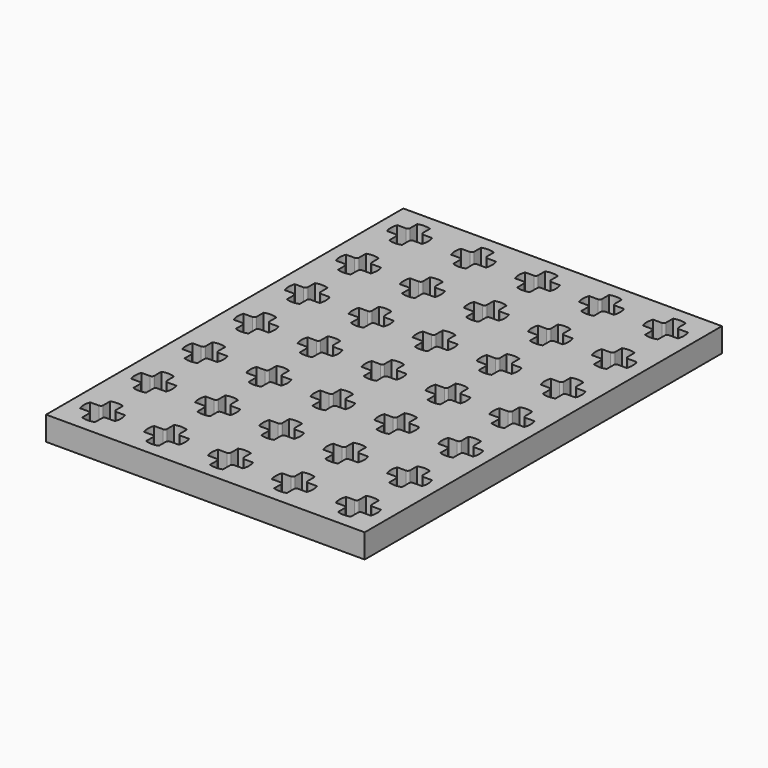
from build123d import *

# Parameters (mm, degrees)
F0_W     = 39.85
F0_H     = 55.85
F1_DEPTH = 3


# Not quite as in the source:
# - a feature names something its author has since deleted; it is built from what else it names


with BuildPart() as f1:
    # F0 (on Top) → F1 (new body)
    with BuildSketch(Plane.XY):
        Rectangle(F0_W, F0_H)
        with BuildLine():
            ThreePointArc((-15.2, -26.1830311496), (-16, -26.325), (-16.8, -26.1830311496))
            Line((-16.8, -26.1830311496), (-16.8, -25.1))
            ThreePointArc((-16.8, -25.1), (-16.8878679656, -24.8878679656), (-17.1, -24.8))
            Line((-17.1, -24.8), (-18.1830311496, -24.8))
            ThreePointArc((-18.1830311496, -24.8), (-18.325, -24), (-18.1830311496, -23.2))
            Line((-18.1830311496, -23.2), (-17.1, -23.2))
            ThreePointArc((-17.1, -23.2), (-16.8878679656, -23.1121320344), (-16.8, -22.9))
            Line((-16.8, -22.9), (-16.8, -21.8169688504))
            ThreePointArc((-16.8, -21.8169688504), (-16, -21.675), (-15.2, -21.8169688504))
            Line((-15.2, -21.8169688504), (-15.2, -22.9))
            ThreePointArc((-15.2, -22.9), (-15.1121320344, -23.1121320344), (-14.9, -23.2))
            Line((-14.9, -23.2), (-13.8169688504, -23.2))
            ThreePointArc((-13.8169688504, -23.2), (-13.675, -24), (-13.8169688504, -24.8))
            Line((-13.8169688504, -24.8), (-14.9, -24.8))
            ThreePointArc((-14.9, -24.8), (-15.1121320344, -24.8878679656), (-15.2, -25.1))
            Line((-15.2, -25.1), (-15.2, -26.1830311496))
        make_face(mode=Mode.SUBTRACT)
        with BuildLine():
            ThreePointArc((-7.2, -26.1830311496), (-8, -26.325), (-8.8, -26.1830311496))
            Line((-8.8, -26.1830311496), (-8.8, -25.1))
            ThreePointArc((-8.8, -25.1), (-8.8878679656, -24.8878679656), (-9.1, -24.8))
            Line((-9.1, -24.8), (-10.1830311496, -24.8))
            ThreePointArc((-10.1830311496, -24.8), (-10.325, -24), (-10.1830311496, -23.2))
            Line((-10.1830311496, -23.2), (-9.1, -23.2))
            ThreePointArc((-9.1, -23.2), (-8.8878679656, -23.1121320344), (-8.8, -22.9))
            Line((-8.8, -22.9), (-8.8, -21.8169688504))
            ThreePointArc((-8.8, -21.8169688504), (-8, -21.675), (-7.2, -21.8169688504))
            Line((-7.2, -21.8169688504), (-7.2, -22.9))
            ThreePointArc((-7.2, -22.9), (-7.1121320344, -23.1121320344), (-6.9, -23.2))
            Line((-6.9, -23.2), (-5.8169688504, -23.2))
            ThreePointArc((-5.8169688504, -23.2), (-5.675, -24), (-5.8169688504, -24.8))
            Line((-5.8169688504, -24.8), (-6.9, -24.8))
            ThreePointArc((-6.9, -24.8), (-7.1121320344, -24.8878679656), (-7.2, -25.1))
            Line((-7.2, -25.1), (-7.2, -26.1830311496))
        make_face(mode=Mode.SUBTRACT)
        with BuildLine():
            ThreePointArc((-15.2, -18.1830311496), (-16, -18.325), (-16.8, -18.1830311496))
            Line((-16.8, -18.1830311496), (-16.8, -17.1))
            ThreePointArc((-16.8, -17.1), (-16.8878679656, -16.8878679656), (-17.1, -16.8))
            Line((-17.1, -16.8), (-18.1830311496, -16.8))
            ThreePointArc((-18.1830311496, -16.8), (-18.325, -16), (-18.1830311496, -15.2))
            Line((-18.1830311496, -15.2), (-17.1, -15.2))
            ThreePointArc((-17.1, -15.2), (-16.8878679656, -15.1121320344), (-16.8, -14.9))
            Line((-16.8, -14.9), (-16.8, -13.8169688504))
            ThreePointArc((-16.8, -13.8169688504), (-16, -13.675), (-15.2, -13.8169688504))
            Line((-15.2, -13.8169688504), (-15.2, -14.9))
            ThreePointArc((-15.2, -14.9), (-15.1121320344, -15.1121320344), (-14.9, -15.2))
            Line((-14.9, -15.2), (-13.8169688504, -15.2))
            ThreePointArc((-13.8169688504, -15.2), (-13.675, -16), (-13.8169688504, -16.8))
            Line((-13.8169688504, -16.8), (-14.9, -16.8))
            ThreePointArc((-14.9, -16.8), (-15.1121320344, -16.8878679656), (-15.2, -17.1))
            Line((-15.2, -17.1), (-15.2, -18.1830311496))
        make_face(mode=Mode.SUBTRACT)
        with BuildLine():
            ThreePointArc((-15.2, -10.1830311496), (-16, -10.325), (-16.8, -10.1830311496))
            Line((-16.8, -10.1830311496), (-16.8, -9.1))
            ThreePointArc((-16.8, -9.1), (-16.8878679656, -8.8878679656), (-17.1, -8.8))
            Line((-17.1, -8.8), (-18.1830311496, -8.8))
            ThreePointArc((-18.1830311496, -8.8), (-18.325, -8), (-18.1830311496, -7.2))
            Line((-18.1830311496, -7.2), (-17.1, -7.2))
            ThreePointArc((-17.1, -7.2), (-16.8878679656, -7.1121320344), (-16.8, -6.9))
            Line((-16.8, -6.9), (-16.8, -5.8169688504))
            ThreePointArc((-16.8, -5.8169688504), (-16, -5.675), (-15.2, -5.8169688504))
            Line((-15.2, -5.8169688504), (-15.2, -6.9))
            ThreePointArc((-15.2, -6.9), (-15.1121320344, -7.1121320344), (-14.9, -7.2))
            Line((-14.9, -7.2), (-13.8169688504, -7.2))
            ThreePointArc((-13.8169688504, -7.2), (-13.675, -8), (-13.8169688504, -8.8))
            Line((-13.8169688504, -8.8), (-14.9, -8.8))
            ThreePointArc((-14.9, -8.8), (-15.1121320344, -8.8878679656), (-15.2, -9.1))
            Line((-15.2, -9.1), (-15.2, -10.1830311496))
        make_face(mode=Mode.SUBTRACT)
        with BuildLine():
            ThreePointArc((-7.2, -18.1830311496), (-8, -18.325), (-8.8, -18.1830311496))
            Line((-8.8, -18.1830311496), (-8.8, -17.1))
            ThreePointArc((-8.8, -17.1), (-8.8878679656, -16.8878679656), (-9.1, -16.8))
            Line((-9.1, -16.8), (-10.1830311496, -16.8))
            ThreePointArc((-10.1830311496, -16.8), (-10.325, -16), (-10.1830311496, -15.2))
            Line((-10.1830311496, -15.2), (-9.1, -15.2))
            ThreePointArc((-9.1, -15.2), (-8.8878679656, -15.1121320344), (-8.8, -14.9))
            Line((-8.8, -14.9), (-8.8, -13.8169688504))
            ThreePointArc((-8.8, -13.8169688504), (-8, -13.675), (-7.2, -13.8169688504))
            Line((-7.2, -13.8169688504), (-7.2, -14.9))
            ThreePointArc((-7.2, -14.9), (-7.1121320344, -15.1121320344), (-6.9, -15.2))
            Line((-6.9, -15.2), (-5.8169688504, -15.2))
            ThreePointArc((-5.8169688504, -15.2), (-5.675, -16), (-5.8169688504, -16.8))
            Line((-5.8169688504, -16.8), (-6.9, -16.8))
            ThreePointArc((-6.9, -16.8), (-7.1121320344, -16.8878679656), (-7.2, -17.1))
            Line((-7.2, -17.1), (-7.2, -18.1830311496))
        make_face(mode=Mode.SUBTRACT)
        with BuildLine():
            ThreePointArc((-7.2, -10.1830311496), (-8, -10.325), (-8.8, -10.1830311496))
            Line((-8.8, -10.1830311496), (-8.8, -9.1))
            ThreePointArc((-8.8, -9.1), (-8.8878679656, -8.8878679656), (-9.1, -8.8))
            Line((-9.1, -8.8), (-10.1830311496, -8.8))
            ThreePointArc((-10.1830311496, -8.8), (-10.325, -8), (-10.1830311496, -7.2))
            Line((-10.1830311496, -7.2), (-9.1, -7.2))
            ThreePointArc((-9.1, -7.2), (-8.8878679656, -7.1121320344), (-8.8, -6.9))
            Line((-8.8, -6.9), (-8.8, -5.8169688504))
            ThreePointArc((-8.8, -5.8169688504), (-8, -5.675), (-7.2, -5.8169688504))
            Line((-7.2, -5.8169688504), (-7.2, -6.9))
            ThreePointArc((-7.2, -6.9), (-7.1121320344, -7.1121320344), (-6.9, -7.2))
            Line((-6.9, -7.2), (-5.8169688504, -7.2))
            ThreePointArc((-5.8169688504, -7.2), (-5.675, -8), (-5.8169688504, -8.8))
            Line((-5.8169688504, -8.8), (-6.9, -8.8))
            ThreePointArc((-6.9, -8.8), (-7.1121320344, -8.8878679656), (-7.2, -9.1))
            Line((-7.2, -9.1), (-7.2, -10.1830311496))
        make_face(mode=Mode.SUBTRACT)
        with BuildLine():
            ThreePointArc((0.8, -26.1830311496), (0, -26.325), (-0.8, -26.1830311496))
            Line((-0.8, -26.1830311496), (-0.8, -25.1))
            ThreePointArc((-0.8, -25.1), (-0.8878679656, -24.8878679656), (-1.1, -24.8))
            Line((-1.1, -24.8), (-2.1830311496, -24.8))
            ThreePointArc((-2.1830311496, -24.8), (-2.325, -24), (-2.1830311496, -23.2))
            Line((-2.1830311496, -23.2), (-1.1, -23.2))
            ThreePointArc((-1.1, -23.2), (-0.8878679656, -23.1121320344), (-0.8, -22.9))
            Line((-0.8, -22.9), (-0.8, -21.8169688504))
            ThreePointArc((-0.8, -21.8169688504), (0, -21.675), (0.8, -21.8169688504))
            Line((0.8, -21.8169688504), (0.8, -22.9))
            ThreePointArc((0.8, -22.9), (0.8878679656, -23.1121320344), (1.1, -23.2))
            Line((1.1, -23.2), (2.1830311496, -23.2))
            ThreePointArc((2.1830311496, -23.2), (2.325, -24), (2.1830311496, -24.8))
            Line((2.1830311496, -24.8), (1.1, -24.8))
            ThreePointArc((1.1, -24.8), (0.8878679656, -24.8878679656), (0.8, -25.1))
            Line((0.8, -25.1), (0.8, -26.1830311496))
        make_face(mode=Mode.SUBTRACT)
        with BuildLine():
            ThreePointArc((8.8, -26.1830311496), (8, -26.325), (7.2, -26.1830311496))
            Line((7.2, -26.1830311496), (7.2, -25.1))
            ThreePointArc((7.2, -25.1), (7.1121320344, -24.8878679656), (6.9, -24.8))
            Line((6.9, -24.8), (5.8169688504, -24.8))
            ThreePointArc((5.8169688504, -24.8), (5.675, -24), (5.8169688504, -23.2))
            Line((5.8169688504, -23.2), (6.9, -23.2))
            ThreePointArc((6.9, -23.2), (7.1121320344, -23.1121320344), (7.2, -22.9))
            Line((7.2, -22.9), (7.2, -21.8169688504))
            ThreePointArc((7.2, -21.8169688504), (8, -21.675), (8.8, -21.8169688504))
            Line((8.8, -21.8169688504), (8.8, -22.9))
            ThreePointArc((8.8, -22.9), (8.8878679656, -23.1121320344), (9.1, -23.2))
            Line((9.1, -23.2), (10.1830311496, -23.2))
            ThreePointArc((10.1830311496, -23.2), (10.325, -24), (10.1830311496, -24.8))
            Line((10.1830311496, -24.8), (9.1, -24.8))
            ThreePointArc((9.1, -24.8), (8.8878679656, -24.8878679656), (8.8, -25.1))
            Line((8.8, -25.1), (8.8, -26.1830311496))
        make_face(mode=Mode.SUBTRACT)
        with BuildLine():
            ThreePointArc((16.8, -26.1830311496), (16, -26.325), (15.2, -26.1830311496))
            Line((15.2, -26.1830311496), (15.2, -25.1))
            ThreePointArc((15.2, -25.1), (15.1121320344, -24.8878679656), (14.9, -24.8))
            Line((14.9, -24.8), (13.8169688504, -24.8))
            ThreePointArc((13.8169688504, -24.8), (13.675, -24), (13.8169688504, -23.2))
            Line((13.8169688504, -23.2), (14.9, -23.2))
            ThreePointArc((14.9, -23.2), (15.1121320344, -23.1121320344), (15.2, -22.9))
            Line((15.2, -22.9), (15.2, -21.8169688504))
            ThreePointArc((15.2, -21.8169688504), (16, -21.675), (16.8, -21.8169688504))
            Line((16.8, -21.8169688504), (16.8, -22.9))
            ThreePointArc((16.8, -22.9), (16.8878679656, -23.1121320344), (17.1, -23.2))
            Line((17.1, -23.2), (18.1830311496, -23.2))
            ThreePointArc((18.1830311496, -23.2), (18.325, -24), (18.1830311496, -24.8))
            Line((18.1830311496, -24.8), (17.1, -24.8))
            ThreePointArc((17.1, -24.8), (16.8878679656, -24.8878679656), (16.8, -25.1))
            Line((16.8, -25.1), (16.8, -26.1830311496))
        make_face(mode=Mode.SUBTRACT)
        with BuildLine():
            ThreePointArc((0.8, -18.1830311496), (0, -18.325), (-0.8, -18.1830311496))
            Line((-0.8, -18.1830311496), (-0.8, -17.1))
            ThreePointArc((-0.8, -17.1), (-0.8878679656, -16.8878679656), (-1.1, -16.8))
            Line((-1.1, -16.8), (-2.1830311496, -16.8))
            ThreePointArc((-2.1830311496, -16.8), (-2.325, -16), (-2.1830311496, -15.2))
            Line((-2.1830311496, -15.2), (-1.1, -15.2))
            ThreePointArc((-1.1, -15.2), (-0.8878679656, -15.1121320344), (-0.8, -14.9))
            Line((-0.8, -14.9), (-0.8, -13.8169688504))
            ThreePointArc((-0.8, -13.8169688504), (0, -13.675), (0.8, -13.8169688504))
            Line((0.8, -13.8169688504), (0.8, -14.9))
            ThreePointArc((0.8, -14.9), (0.8878679656, -15.1121320344), (1.1, -15.2))
            Line((1.1, -15.2), (2.1830311496, -15.2))
            ThreePointArc((2.1830311496, -15.2), (2.325, -16), (2.1830311496, -16.8))
            Line((2.1830311496, -16.8), (1.1, -16.8))
            ThreePointArc((1.1, -16.8), (0.8878679656, -16.8878679656), (0.8, -17.1))
            Line((0.8, -17.1), (0.8, -18.1830311496))
        make_face(mode=Mode.SUBTRACT)
        with BuildLine():
            ThreePointArc((8.8, -18.1830311496), (8, -18.325), (7.2, -18.1830311496))
            Line((7.2, -18.1830311496), (7.2, -17.1))
            ThreePointArc((7.2, -17.1), (7.1121320344, -16.8878679656), (6.9, -16.8))
            Line((6.9, -16.8), (5.8169688504, -16.8))
            ThreePointArc((5.8169688504, -16.8), (5.675, -16), (5.8169688504, -15.2))
            Line((5.8169688504, -15.2), (6.9, -15.2))
            ThreePointArc((6.9, -15.2), (7.1121320344, -15.1121320344), (7.2, -14.9))
            Line((7.2, -14.9), (7.2, -13.8169688504))
            ThreePointArc((7.2, -13.8169688504), (8, -13.675), (8.8, -13.8169688504))
            Line((8.8, -13.8169688504), (8.8, -14.9))
            ThreePointArc((8.8, -14.9), (8.8878679656, -15.1121320344), (9.1, -15.2))
            Line((9.1, -15.2), (10.1830311496, -15.2))
            ThreePointArc((10.1830311496, -15.2), (10.325, -16), (10.1830311496, -16.8))
            Line((10.1830311496, -16.8), (9.1, -16.8))
            ThreePointArc((9.1, -16.8), (8.8878679656, -16.8878679656), (8.8, -17.1))
            Line((8.8, -17.1), (8.8, -18.1830311496))
        make_face(mode=Mode.SUBTRACT)
        with BuildLine():
            ThreePointArc((0.8, -10.1830311496), (0, -10.325), (-0.8, -10.1830311496))
            Line((-0.8, -10.1830311496), (-0.8, -9.1))
            ThreePointArc((-0.8, -9.1), (-0.8878679656, -8.8878679656), (-1.1, -8.8))
            Line((-1.1, -8.8), (-2.1830311496, -8.8))
            ThreePointArc((-2.1830311496, -8.8), (-2.325, -8), (-2.1830311496, -7.2))
            Line((-2.1830311496, -7.2), (-1.1, -7.2))
            ThreePointArc((-1.1, -7.2), (-0.8878679656, -7.1121320344), (-0.8, -6.9))
            Line((-0.8, -6.9), (-0.8, -5.8169688504))
            ThreePointArc((-0.8, -5.8169688504), (0, -5.675), (0.8, -5.8169688504))
            Line((0.8, -5.8169688504), (0.8, -6.9))
            ThreePointArc((0.8, -6.9), (0.8878679656, -7.1121320344), (1.1, -7.2))
            Line((1.1, -7.2), (2.1830311496, -7.2))
            ThreePointArc((2.1830311496, -7.2), (2.325, -8), (2.1830311496, -8.8))
            Line((2.1830311496, -8.8), (1.1, -8.8))
            ThreePointArc((1.1, -8.8), (0.8878679656, -8.8878679656), (0.8, -9.1))
            Line((0.8, -9.1), (0.8, -10.1830311496))
        make_face(mode=Mode.SUBTRACT)
        with BuildLine():
            ThreePointArc((8.8, -10.1830311496), (8, -10.325), (7.2, -10.1830311496))
            Line((7.2, -10.1830311496), (7.2, -9.1))
            ThreePointArc((7.2, -9.1), (7.1121320344, -8.8878679656), (6.9, -8.8))
            Line((6.9, -8.8), (5.8169688504, -8.8))
            ThreePointArc((5.8169688504, -8.8), (5.675, -8), (5.8169688504, -7.2))
            Line((5.8169688504, -7.2), (6.9, -7.2))
            ThreePointArc((6.9, -7.2), (7.1121320344, -7.1121320344), (7.2, -6.9))
            Line((7.2, -6.9), (7.2, -5.8169688504))
            ThreePointArc((7.2, -5.8169688504), (8, -5.675), (8.8, -5.8169688504))
            Line((8.8, -5.8169688504), (8.8, -6.9))
            ThreePointArc((8.8, -6.9), (8.8878679656, -7.1121320344), (9.1, -7.2))
            Line((9.1, -7.2), (10.1830311496, -7.2))
            ThreePointArc((10.1830311496, -7.2), (10.325, -8), (10.1830311496, -8.8))
            Line((10.1830311496, -8.8), (9.1, -8.8))
            ThreePointArc((9.1, -8.8), (8.8878679656, -8.8878679656), (8.8, -9.1))
            Line((8.8, -9.1), (8.8, -10.1830311496))
        make_face(mode=Mode.SUBTRACT)
        with BuildLine():
            ThreePointArc((16.8, -18.1830311496), (16, -18.325), (15.2, -18.1830311496))
            Line((15.2, -18.1830311496), (15.2, -17.1))
            ThreePointArc((15.2, -17.1), (15.1121320344, -16.8878679656), (14.9, -16.8))
            Line((14.9, -16.8), (13.8169688504, -16.8))
            ThreePointArc((13.8169688504, -16.8), (13.675, -16), (13.8169688504, -15.2))
            Line((13.8169688504, -15.2), (14.9, -15.2))
            ThreePointArc((14.9, -15.2), (15.1121320344, -15.1121320344), (15.2, -14.9))
            Line((15.2, -14.9), (15.2, -13.8169688504))
            ThreePointArc((15.2, -13.8169688504), (16, -13.675), (16.8, -13.8169688504))
            Line((16.8, -13.8169688504), (16.8, -14.9))
            ThreePointArc((16.8, -14.9), (16.8878679656, -15.1121320344), (17.1, -15.2))
            Line((17.1, -15.2), (18.1830311496, -15.2))
            ThreePointArc((18.1830311496, -15.2), (18.325, -16), (18.1830311496, -16.8))
            Line((18.1830311496, -16.8), (17.1, -16.8))
            ThreePointArc((17.1, -16.8), (16.8878679656, -16.8878679656), (16.8, -17.1))
            Line((16.8, -17.1), (16.8, -18.1830311496))
        make_face(mode=Mode.SUBTRACT)
        with BuildLine():
            ThreePointArc((16.8, -10.1830311496), (16, -10.325), (15.2, -10.1830311496))
            Line((15.2, -10.1830311496), (15.2, -9.1))
            ThreePointArc((15.2, -9.1), (15.1121320344, -8.8878679656), (14.9, -8.8))
            Line((14.9, -8.8), (13.8169688504, -8.8))
            ThreePointArc((13.8169688504, -8.8), (13.675, -8), (13.8169688504, -7.2))
            Line((13.8169688504, -7.2), (14.9, -7.2))
            ThreePointArc((14.9, -7.2), (15.1121320344, -7.1121320344), (15.2, -6.9))
            Line((15.2, -6.9), (15.2, -5.8169688504))
            ThreePointArc((15.2, -5.8169688504), (16, -5.675), (16.8, -5.8169688504))
            Line((16.8, -5.8169688504), (16.8, -6.9))
            ThreePointArc((16.8, -6.9), (16.8878679656, -7.1121320344), (17.1, -7.2))
            Line((17.1, -7.2), (18.1830311496, -7.2))
            ThreePointArc((18.1830311496, -7.2), (18.325, -8), (18.1830311496, -8.8))
            Line((18.1830311496, -8.8), (17.1, -8.8))
            ThreePointArc((17.1, -8.8), (16.8878679656, -8.8878679656), (16.8, -9.1))
            Line((16.8, -9.1), (16.8, -10.1830311496))
        make_face(mode=Mode.SUBTRACT)
        with BuildLine():
            ThreePointArc((-15.2, -2.1830311496), (-16, -2.325), (-16.8, -2.1830311496))
            Line((-16.8, -2.1830311496), (-16.8, -1.1))
            ThreePointArc((-16.8, -1.1), (-16.8878679656, -0.8878679656), (-17.1, -0.8))
            Line((-17.1, -0.8), (-18.1830311496, -0.8))
            ThreePointArc((-18.1830311496, -0.8), (-18.325, 0), (-18.1830311496, 0.8))
            Line((-18.1830311496, 0.8), (-17.1, 0.8))
            ThreePointArc((-17.1, 0.8), (-16.8878679656, 0.8878679656), (-16.8, 1.1))
            Line((-16.8, 1.1), (-16.8, 2.1830311496))
            ThreePointArc((-16.8, 2.1830311496), (-16, 2.325), (-15.2, 2.1830311496))
            Line((-15.2, 2.1830311496), (-15.2, 1.1))
            ThreePointArc((-15.2, 1.1), (-15.1121320344, 0.8878679656), (-14.9, 0.8))
            Line((-14.9, 0.8), (-13.8169688504, 0.8))
            ThreePointArc((-13.8169688504, 0.8), (-13.675, 0), (-13.8169688504, -0.8))
            Line((-13.8169688504, -0.8), (-14.9, -0.8))
            ThreePointArc((-14.9, -0.8), (-15.1121320344, -0.8878679656), (-15.2, -1.1))
            Line((-15.2, -1.1), (-15.2, -2.1830311496))
        make_face(mode=Mode.SUBTRACT)
        with BuildLine():
            ThreePointArc((-15.2, 5.8169688504), (-16, 5.675), (-16.8, 5.8169688504))
            Line((-16.8, 5.8169688504), (-16.8, 6.9))
            ThreePointArc((-16.8, 6.9), (-16.8878679656, 7.1121320344), (-17.1, 7.2))
            Line((-17.1, 7.2), (-18.1830311496, 7.2))
            ThreePointArc((-18.1830311496, 7.2), (-18.325, 8), (-18.1830311496, 8.8))
            Line((-18.1830311496, 8.8), (-17.1, 8.8))
            ThreePointArc((-17.1, 8.8), (-16.8878679656, 8.8878679656), (-16.8, 9.1))
            Line((-16.8, 9.1), (-16.8, 10.1830311496))
            ThreePointArc((-16.8, 10.1830311496), (-16, 10.325), (-15.2, 10.1830311496))
            Line((-15.2, 10.1830311496), (-15.2, 9.1))
            ThreePointArc((-15.2, 9.1), (-15.1121320344, 8.8878679656), (-14.9, 8.8))
            Line((-14.9, 8.8), (-13.8169688504, 8.8))
            ThreePointArc((-13.8169688504, 8.8), (-13.675, 8), (-13.8169688504, 7.2))
            Line((-13.8169688504, 7.2), (-14.9, 7.2))
            ThreePointArc((-14.9, 7.2), (-15.1121320344, 7.1121320344), (-15.2, 6.9))
            Line((-15.2, 6.9), (-15.2, 5.8169688504))
        make_face(mode=Mode.SUBTRACT)
        with BuildLine():
            ThreePointArc((-7.2, -2.1830311496), (-8, -2.325), (-8.8, -2.1830311496))
            Line((-8.8, -2.1830311496), (-8.8, -1.1))
            ThreePointArc((-8.8, -1.1), (-8.8878679656, -0.8878679656), (-9.1, -0.8))
            Line((-9.1, -0.8), (-10.1830311496, -0.8))
            ThreePointArc((-10.1830311496, -0.8), (-10.325, 0), (-10.1830311496, 0.8))
            Line((-10.1830311496, 0.8), (-9.1, 0.8))
            ThreePointArc((-9.1, 0.8), (-8.8878679656, 0.8878679656), (-8.8, 1.1))
            Line((-8.8, 1.1), (-8.8, 2.1830311496))
            ThreePointArc((-8.8, 2.1830311496), (-8, 2.325), (-7.2, 2.1830311496))
            Line((-7.2, 2.1830311496), (-7.2, 1.1))
            ThreePointArc((-7.2, 1.1), (-7.1121320344, 0.8878679656), (-6.9, 0.8))
            Line((-6.9, 0.8), (-5.8169688504, 0.8))
            ThreePointArc((-5.8169688504, 0.8), (-5.675, 0), (-5.8169688504, -0.8))
            Line((-5.8169688504, -0.8), (-6.9, -0.8))
            ThreePointArc((-6.9, -0.8), (-7.1121320344, -0.8878679656), (-7.2, -1.1))
            Line((-7.2, -1.1), (-7.2, -2.1830311496))
        make_face(mode=Mode.SUBTRACT)
        with BuildLine():
            ThreePointArc((-7.2, 5.8169688504), (-8, 5.675), (-8.8, 5.8169688504))
            Line((-8.8, 5.8169688504), (-8.8, 6.9))
            ThreePointArc((-8.8, 6.9), (-8.8878679656, 7.1121320344), (-9.1, 7.2))
            Line((-9.1, 7.2), (-10.1830311496, 7.2))
            ThreePointArc((-10.1830311496, 7.2), (-10.325, 8), (-10.1830311496, 8.8))
            Line((-10.1830311496, 8.8), (-9.1, 8.8))
            ThreePointArc((-9.1, 8.8), (-8.8878679656, 8.8878679656), (-8.8, 9.1))
            Line((-8.8, 9.1), (-8.8, 10.1830311496))
            ThreePointArc((-8.8, 10.1830311496), (-8, 10.325), (-7.2, 10.1830311496))
            Line((-7.2, 10.1830311496), (-7.2, 9.1))
            ThreePointArc((-7.2, 9.1), (-7.1121320344, 8.8878679656), (-6.9, 8.8))
            Line((-6.9, 8.8), (-5.8169688504, 8.8))
            ThreePointArc((-5.8169688504, 8.8), (-5.675, 8), (-5.8169688504, 7.2))
            Line((-5.8169688504, 7.2), (-6.9, 7.2))
            ThreePointArc((-6.9, 7.2), (-7.1121320344, 7.1121320344), (-7.2, 6.9))
            Line((-7.2, 6.9), (-7.2, 5.8169688504))
        make_face(mode=Mode.SUBTRACT)
        with BuildLine():
            ThreePointArc((-15.2, 13.8169688504), (-16, 13.675), (-16.8, 13.8169688504))
            Line((-16.8, 13.8169688504), (-16.8, 14.9))
            ThreePointArc((-16.8, 14.9), (-16.8878679656, 15.1121320344), (-17.1, 15.2))
            Line((-17.1, 15.2), (-18.1830311496, 15.2))
            ThreePointArc((-18.1830311496, 15.2), (-18.325, 16), (-18.1830311496, 16.8))
            Line((-18.1830311496, 16.8), (-17.1, 16.8))
            ThreePointArc((-17.1, 16.8), (-16.8878679656, 16.8878679656), (-16.8, 17.1))
            Line((-16.8, 17.1), (-16.8, 18.1830311496))
            ThreePointArc((-16.8, 18.1830311496), (-16, 18.325), (-15.2, 18.1830311496))
            Line((-15.2, 18.1830311496), (-15.2, 17.1))
            ThreePointArc((-15.2, 17.1), (-15.1121320344, 16.8878679656), (-14.9, 16.8))
            Line((-14.9, 16.8), (-13.8169688504, 16.8))
            ThreePointArc((-13.8169688504, 16.8), (-13.675, 16), (-13.8169688504, 15.2))
            Line((-13.8169688504, 15.2), (-14.9, 15.2))
            ThreePointArc((-14.9, 15.2), (-15.1121320344, 15.1121320344), (-15.2, 14.9))
            Line((-15.2, 14.9), (-15.2, 13.8169688504))
        make_face(mode=Mode.SUBTRACT)
        with BuildLine():
            ThreePointArc((-16.8, 26.1830311496), (-16, 26.325), (-15.2, 26.1830311496))
            Line((-15.2, 26.1830311496), (-15.2, 25.1))
            ThreePointArc((-15.2, 25.1), (-15.1121320344, 24.8878679656), (-14.9, 24.8))
            Line((-14.9, 24.8), (-13.8169688504, 24.8))
            ThreePointArc((-13.8169688504, 24.8), (-13.675, 24), (-13.8169688504, 23.2))
            Line((-13.8169688504, 23.2), (-14.9, 23.2))
            ThreePointArc((-14.9, 23.2), (-15.1121320344, 23.1121320344), (-15.2, 22.9))
            Line((-15.2, 22.9), (-15.2, 21.8169688504))
            ThreePointArc((-15.2, 21.8169688504), (-16, 21.675), (-16.8, 21.8169688504))
            Line((-16.8, 21.8169688504), (-16.8, 22.9))
            ThreePointArc((-16.8, 22.9), (-16.8878679656, 23.1121320344), (-17.1, 23.2))
            Line((-17.1, 23.2), (-18.1830311496, 23.2))
            ThreePointArc((-18.1830311496, 23.2), (-18.325, 24), (-18.1830311496, 24.8))
            Line((-18.1830311496, 24.8), (-17.1, 24.8))
            ThreePointArc((-17.1, 24.8), (-16.8878679656, 24.8878679656), (-16.8, 25.1))
            Line((-16.8, 25.1), (-16.8, 26.1830311496))
        make_face(mode=Mode.SUBTRACT)
        with BuildLine():
            ThreePointArc((-7.2, 13.8169688504), (-8, 13.675), (-8.8, 13.8169688504))
            Line((-8.8, 13.8169688504), (-8.8, 14.9))
            ThreePointArc((-8.8, 14.9), (-8.8878679656, 15.1121320344), (-9.1, 15.2))
            Line((-9.1, 15.2), (-10.1830311496, 15.2))
            ThreePointArc((-10.1830311496, 15.2), (-10.325, 16), (-10.1830311496, 16.8))
            Line((-10.1830311496, 16.8), (-9.1, 16.8))
            ThreePointArc((-9.1, 16.8), (-8.8878679656, 16.8878679656), (-8.8, 17.1))
            Line((-8.8, 17.1), (-8.8, 18.1830311496))
            ThreePointArc((-8.8, 18.1830311496), (-8, 18.325), (-7.2, 18.1830311496))
            Line((-7.2, 18.1830311496), (-7.2, 17.1))
            ThreePointArc((-7.2, 17.1), (-7.1121320344, 16.8878679656), (-6.9, 16.8))
            Line((-6.9, 16.8), (-5.8169688504, 16.8))
            ThreePointArc((-5.8169688504, 16.8), (-5.675, 16), (-5.8169688504, 15.2))
            Line((-5.8169688504, 15.2), (-6.9, 15.2))
            ThreePointArc((-6.9, 15.2), (-7.1121320344, 15.1121320344), (-7.2, 14.9))
            Line((-7.2, 14.9), (-7.2, 13.8169688504))
        make_face(mode=Mode.SUBTRACT)
        with BuildLine():
            ThreePointArc((-7.2, 21.8169688504), (-8, 21.675), (-8.8, 21.8169688504))
            Line((-8.8, 21.8169688504), (-8.8, 22.9))
            ThreePointArc((-8.8, 22.9), (-8.8878679656, 23.1121320344), (-9.1, 23.2))
            Line((-9.1, 23.2), (-10.1830311496, 23.2))
            ThreePointArc((-10.1830311496, 23.2), (-10.325, 24), (-10.1830311496, 24.8))
            Line((-10.1830311496, 24.8), (-9.1, 24.8))
            ThreePointArc((-9.1, 24.8), (-8.8878679656, 24.8878679656), (-8.8, 25.1))
            Line((-8.8, 25.1), (-8.8, 26.1830311496))
            ThreePointArc((-8.8, 26.1830311496), (-8, 26.325), (-7.2, 26.1830311496))
            Line((-7.2, 26.1830311496), (-7.2, 25.1))
            ThreePointArc((-7.2, 25.1), (-7.1121320344, 24.8878679656), (-6.9, 24.8))
            Line((-6.9, 24.8), (-5.8169688504, 24.8))
            ThreePointArc((-5.8169688504, 24.8), (-5.675, 24), (-5.8169688504, 23.2))
            Line((-5.8169688504, 23.2), (-6.9, 23.2))
            ThreePointArc((-6.9, 23.2), (-7.1121320344, 23.1121320344), (-7.2, 22.9))
            Line((-7.2, 22.9), (-7.2, 21.8169688504))
        make_face(mode=Mode.SUBTRACT)
        with BuildLine():
            ThreePointArc((0.8, -2.1830311496), (0, -2.325), (-0.8, -2.1830311496))
            Line((-0.8, -2.1830311496), (-0.8, -1.1))
            ThreePointArc((-0.8, -1.1), (-0.8878679656, -0.8878679656), (-1.1, -0.8))
            Line((-1.1, -0.8), (-2.1830311496, -0.8))
            ThreePointArc((-2.1830311496, -0.8), (-2.325, 0), (-2.1830311496, 0.8))
            Line((-2.1830311496, 0.8), (-1.1, 0.8))
            ThreePointArc((-1.1, 0.8), (-0.8878679656, 0.8878679656), (-0.8, 1.1))
            Line((-0.8, 1.1), (-0.8, 2.1830311496))
            ThreePointArc((-0.8, 2.1830311496), (0, 2.325), (0.8, 2.1830311496))
            Line((0.8, 2.1830311496), (0.8, 1.1))
            ThreePointArc((0.8, 1.1), (0.8878679656, 0.8878679656), (1.1, 0.8))
            Line((1.1, 0.8), (2.1830311496, 0.8))
            ThreePointArc((2.1830311496, 0.8), (2.325, 0), (2.1830311496, -0.8))
            Line((2.1830311496, -0.8), (1.1, -0.8))
            ThreePointArc((1.1, -0.8), (0.8878679656, -0.8878679656), (0.8, -1.1))
            Line((0.8, -1.1), (0.8, -2.1830311496))
        make_face(mode=Mode.SUBTRACT)
        with BuildLine():
            ThreePointArc((8.8, -2.1830311496), (8, -2.325), (7.2, -2.1830311496))
            Line((7.2, -2.1830311496), (7.2, -1.1))
            ThreePointArc((7.2, -1.1), (7.1121320344, -0.8878679656), (6.9, -0.8))
            Line((6.9, -0.8), (5.8169688504, -0.8))
            ThreePointArc((5.8169688504, -0.8), (5.675, 0), (5.8169688504, 0.8))
            Line((5.8169688504, 0.8), (6.9, 0.8))
            ThreePointArc((6.9, 0.8), (7.1121320344, 0.8878679656), (7.2, 1.1))
            Line((7.2, 1.1), (7.2, 2.1830311496))
            ThreePointArc((7.2, 2.1830311496), (8, 2.325), (8.8, 2.1830311496))
            Line((8.8, 2.1830311496), (8.8, 1.1))
            ThreePointArc((8.8, 1.1), (8.8878679656, 0.8878679656), (9.1, 0.8))
            Line((9.1, 0.8), (10.1830311496, 0.8))
            ThreePointArc((10.1830311496, 0.8), (10.325, 0), (10.1830311496, -0.8))
            Line((10.1830311496, -0.8), (9.1, -0.8))
            ThreePointArc((9.1, -0.8), (8.8878679656, -0.8878679656), (8.8, -1.1))
            Line((8.8, -1.1), (8.8, -2.1830311496))
        make_face(mode=Mode.SUBTRACT)
        with BuildLine():
            ThreePointArc((0.8, 5.8169688504), (0, 5.675), (-0.8, 5.8169688504))
            Line((-0.8, 5.8169688504), (-0.8, 6.9))
            ThreePointArc((-0.8, 6.9), (-0.8878679656, 7.1121320344), (-1.1, 7.2))
            Line((-1.1, 7.2), (-2.1830311496, 7.2))
            ThreePointArc((-2.1830311496, 7.2), (-2.325, 8), (-2.1830311496, 8.8))
            Line((-2.1830311496, 8.8), (-1.1, 8.8))
            ThreePointArc((-1.1, 8.8), (-0.8878679656, 8.8878679656), (-0.8, 9.1))
            Line((-0.8, 9.1), (-0.8, 10.1830311496))
            ThreePointArc((-0.8, 10.1830311496), (0, 10.325), (0.8, 10.1830311496))
            Line((0.8, 10.1830311496), (0.8, 9.1))
            ThreePointArc((0.8, 9.1), (0.8878679656, 8.8878679656), (1.1, 8.8))
            Line((1.1, 8.8), (2.1830311496, 8.8))
            ThreePointArc((2.1830311496, 8.8), (2.325, 8), (2.1830311496, 7.2))
            Line((2.1830311496, 7.2), (1.1, 7.2))
            ThreePointArc((1.1, 7.2), (0.8878679656, 7.1121320344), (0.8, 6.9))
            Line((0.8, 6.9), (0.8, 5.8169688504))
        make_face(mode=Mode.SUBTRACT)
        with BuildLine():
            ThreePointArc((8.8, 5.8169688504), (8, 5.675), (7.2, 5.8169688504))
            Line((7.2, 5.8169688504), (7.2, 6.9))
            ThreePointArc((7.2, 6.9), (7.1121320344, 7.1121320344), (6.9, 7.2))
            Line((6.9, 7.2), (5.8169688504, 7.2))
            ThreePointArc((5.8169688504, 7.2), (5.675, 8), (5.8169688504, 8.8))
            Line((5.8169688504, 8.8), (6.9, 8.8))
            ThreePointArc((6.9, 8.8), (7.1121320344, 8.8878679656), (7.2, 9.1))
            Line((7.2, 9.1), (7.2, 10.1830311496))
            ThreePointArc((7.2, 10.1830311496), (8, 10.325), (8.8, 10.1830311496))
            Line((8.8, 10.1830311496), (8.8, 9.1))
            ThreePointArc((8.8, 9.1), (8.8878679656, 8.8878679656), (9.1, 8.8))
            Line((9.1, 8.8), (10.1830311496, 8.8))
            ThreePointArc((10.1830311496, 8.8), (10.325, 8), (10.1830311496, 7.2))
            Line((10.1830311496, 7.2), (9.1, 7.2))
            ThreePointArc((9.1, 7.2), (8.8878679656, 7.1121320344), (8.8, 6.9))
            Line((8.8, 6.9), (8.8, 5.8169688504))
        make_face(mode=Mode.SUBTRACT)
        with BuildLine():
            ThreePointArc((16.8, -2.1830311496), (16, -2.325), (15.2, -2.1830311496))
            Line((15.2, -2.1830311496), (15.2, -1.1))
            ThreePointArc((15.2, -1.1), (15.1121320344, -0.8878679656), (14.9, -0.8))
            Line((14.9, -0.8), (13.8169688504, -0.8))
            ThreePointArc((13.8169688504, -0.8), (13.675, 0), (13.8169688504, 0.8))
            Line((13.8169688504, 0.8), (14.9, 0.8))
            ThreePointArc((14.9, 0.8), (15.1121320344, 0.8878679656), (15.2, 1.1))
            Line((15.2, 1.1), (15.2, 2.1830311496))
            ThreePointArc((15.2, 2.1830311496), (16, 2.325), (16.8, 2.1830311496))
            Line((16.8, 2.1830311496), (16.8, 1.1))
            ThreePointArc((16.8, 1.1), (16.8878679656, 0.8878679656), (17.1, 0.8))
            Line((17.1, 0.8), (18.1830311496, 0.8))
            ThreePointArc((18.1830311496, 0.8), (18.325, 0), (18.1830311496, -0.8))
            Line((18.1830311496, -0.8), (17.1, -0.8))
            ThreePointArc((17.1, -0.8), (16.8878679656, -0.8878679656), (16.8, -1.1))
            Line((16.8, -1.1), (16.8, -2.1830311496))
        make_face(mode=Mode.SUBTRACT)
        with BuildLine():
            ThreePointArc((16.8, 5.8169688504), (16, 5.675), (15.2, 5.8169688504))
            Line((15.2, 5.8169688504), (15.2, 6.9))
            ThreePointArc((15.2, 6.9), (15.1121320344, 7.1121320344), (14.9, 7.2))
            Line((14.9, 7.2), (13.8169688504, 7.2))
            ThreePointArc((13.8169688504, 7.2), (13.675, 8), (13.8169688504, 8.8))
            Line((13.8169688504, 8.8), (14.9, 8.8))
            ThreePointArc((14.9, 8.8), (15.1121320344, 8.8878679656), (15.2, 9.1))
            Line((15.2, 9.1), (15.2, 10.1830311496))
            ThreePointArc((15.2, 10.1830311496), (16, 10.325), (16.8, 10.1830311496))
            Line((16.8, 10.1830311496), (16.8, 9.1))
            ThreePointArc((16.8, 9.1), (16.8878679656, 8.8878679656), (17.1, 8.8))
            Line((17.1, 8.8), (18.1830311496, 8.8))
            ThreePointArc((18.1830311496, 8.8), (18.325, 8), (18.1830311496, 7.2))
            Line((18.1830311496, 7.2), (17.1, 7.2))
            ThreePointArc((17.1, 7.2), (16.8878679656, 7.1121320344), (16.8, 6.9))
            Line((16.8, 6.9), (16.8, 5.8169688504))
        make_face(mode=Mode.SUBTRACT)
        with BuildLine():
            ThreePointArc((0.8, 13.8169688504), (0, 13.675), (-0.8, 13.8169688504))
            Line((-0.8, 13.8169688504), (-0.8, 14.9))
            ThreePointArc((-0.8, 14.9), (-0.8878679656, 15.1121320344), (-1.1, 15.2))
            Line((-1.1, 15.2), (-2.1830311496, 15.2))
            ThreePointArc((-2.1830311496, 15.2), (-2.325, 16), (-2.1830311496, 16.8))
            Line((-2.1830311496, 16.8), (-1.1, 16.8))
            ThreePointArc((-1.1, 16.8), (-0.8878679656, 16.8878679656), (-0.8, 17.1))
            Line((-0.8, 17.1), (-0.8, 18.1830311496))
            ThreePointArc((-0.8, 18.1830311496), (0, 18.325), (0.8, 18.1830311496))
            Line((0.8, 18.1830311496), (0.8, 17.1))
            ThreePointArc((0.8, 17.1), (0.8878679656, 16.8878679656), (1.1, 16.8))
            Line((1.1, 16.8), (2.1830311496, 16.8))
            ThreePointArc((2.1830311496, 16.8), (2.325, 16), (2.1830311496, 15.2))
            Line((2.1830311496, 15.2), (1.1, 15.2))
            ThreePointArc((1.1, 15.2), (0.8878679656, 15.1121320344), (0.8, 14.9))
            Line((0.8, 14.9), (0.8, 13.8169688504))
        make_face(mode=Mode.SUBTRACT)
        with BuildLine():
            ThreePointArc((8.8, 13.8169688504), (8, 13.675), (7.2, 13.8169688504))
            Line((7.2, 13.8169688504), (7.2, 14.9))
            ThreePointArc((7.2, 14.9), (7.1121320344, 15.1121320344), (6.9, 15.2))
            Line((6.9, 15.2), (5.8169688504, 15.2))
            ThreePointArc((5.8169688504, 15.2), (5.675, 16), (5.8169688504, 16.8))
            Line((5.8169688504, 16.8), (6.9, 16.8))
            ThreePointArc((6.9, 16.8), (7.1121320344, 16.8878679656), (7.2, 17.1))
            Line((7.2, 17.1), (7.2, 18.1830311496))
            ThreePointArc((7.2, 18.1830311496), (8, 18.325), (8.8, 18.1830311496))
            Line((8.8, 18.1830311496), (8.8, 17.1))
            ThreePointArc((8.8, 17.1), (8.8878679656, 16.8878679656), (9.1, 16.8))
            Line((9.1, 16.8), (10.1830311496, 16.8))
            ThreePointArc((10.1830311496, 16.8), (10.325, 16), (10.1830311496, 15.2))
            Line((10.1830311496, 15.2), (9.1, 15.2))
            ThreePointArc((9.1, 15.2), (8.8878679656, 15.1121320344), (8.8, 14.9))
            Line((8.8, 14.9), (8.8, 13.8169688504))
        make_face(mode=Mode.SUBTRACT)
        with BuildLine():
            ThreePointArc((0.8, 21.8169688504), (0, 21.675), (-0.8, 21.8169688504))
            Line((-0.8, 21.8169688504), (-0.8, 22.9))
            ThreePointArc((-0.8, 22.9), (-0.8878679656, 23.1121320344), (-1.1, 23.2))
            Line((-1.1, 23.2), (-2.1830311496, 23.2))
            ThreePointArc((-2.1830311496, 23.2), (-2.325, 24), (-2.1830311496, 24.8))
            Line((-2.1830311496, 24.8), (-1.1, 24.8))
            ThreePointArc((-1.1, 24.8), (-0.8878679656, 24.8878679656), (-0.8, 25.1))
            Line((-0.8, 25.1), (-0.8, 26.1830311496))
            ThreePointArc((-0.8, 26.1830311496), (0, 26.325), (0.8, 26.1830311496))
            Line((0.8, 26.1830311496), (0.8, 25.1))
            ThreePointArc((0.8, 25.1), (0.8878679656, 24.8878679656), (1.1, 24.8))
            Line((1.1, 24.8), (2.1830311496, 24.8))
            ThreePointArc((2.1830311496, 24.8), (2.325, 24), (2.1830311496, 23.2))
            Line((2.1830311496, 23.2), (1.1, 23.2))
            ThreePointArc((1.1, 23.2), (0.8878679656, 23.1121320344), (0.8, 22.9))
            Line((0.8, 22.9), (0.8, 21.8169688504))
        make_face(mode=Mode.SUBTRACT)
        with BuildLine():
            ThreePointArc((8.8, 21.8169688504), (8, 21.675), (7.2, 21.8169688504))
            Line((7.2, 21.8169688504), (7.2, 22.9))
            ThreePointArc((7.2, 22.9), (7.1121320344, 23.1121320344), (6.9, 23.2))
            Line((6.9, 23.2), (5.8169688504, 23.2))
            ThreePointArc((5.8169688504, 23.2), (5.675, 24), (5.8169688504, 24.8))
            Line((5.8169688504, 24.8), (6.9, 24.8))
            ThreePointArc((6.9, 24.8), (7.1121320344, 24.8878679656), (7.2, 25.1))
            Line((7.2, 25.1), (7.2, 26.1830311496))
            ThreePointArc((7.2, 26.1830311496), (8, 26.325), (8.8, 26.1830311496))
            Line((8.8, 26.1830311496), (8.8, 25.1))
            ThreePointArc((8.8, 25.1), (8.8878679656, 24.8878679656), (9.1, 24.8))
            Line((9.1, 24.8), (10.1830311496, 24.8))
            ThreePointArc((10.1830311496, 24.8), (10.325, 24), (10.1830311496, 23.2))
            Line((10.1830311496, 23.2), (9.1, 23.2))
            ThreePointArc((9.1, 23.2), (8.8878679656, 23.1121320344), (8.8, 22.9))
            Line((8.8, 22.9), (8.8, 21.8169688504))
        make_face(mode=Mode.SUBTRACT)
        with BuildLine():
            ThreePointArc((16.8, 13.8169688504), (16, 13.675), (15.2, 13.8169688504))
            Line((15.2, 13.8169688504), (15.2, 14.9))
            ThreePointArc((15.2, 14.9), (15.1121320344, 15.1121320344), (14.9, 15.2))
            Line((14.9, 15.2), (13.8169688504, 15.2))
            ThreePointArc((13.8169688504, 15.2), (13.675, 16), (13.8169688504, 16.8))
            Line((13.8169688504, 16.8), (14.9, 16.8))
            ThreePointArc((14.9, 16.8), (15.1121320344, 16.8878679656), (15.2, 17.1))
            Line((15.2, 17.1), (15.2, 18.1830311496))
            ThreePointArc((15.2, 18.1830311496), (16, 18.325), (16.8, 18.1830311496))
            Line((16.8, 18.1830311496), (16.8, 17.1))
            ThreePointArc((16.8, 17.1), (16.8878679656, 16.8878679656), (17.1, 16.8))
            Line((17.1, 16.8), (18.1830311496, 16.8))
            ThreePointArc((18.1830311496, 16.8), (18.325, 16), (18.1830311496, 15.2))
            Line((18.1830311496, 15.2), (17.1, 15.2))
            ThreePointArc((17.1, 15.2), (16.8878679656, 15.1121320344), (16.8, 14.9))
            Line((16.8, 14.9), (16.8, 13.8169688504))
        make_face(mode=Mode.SUBTRACT)
        with BuildLine():
            ThreePointArc((16.8, 21.8169688504), (16, 21.675), (15.2, 21.8169688504))
            Line((15.2, 21.8169688504), (15.2, 22.9))
            ThreePointArc((15.2, 22.9), (15.1121320344, 23.1121320344), (14.9, 23.2))
            Line((14.9, 23.2), (13.8169688504, 23.2))
            ThreePointArc((13.8169688504, 23.2), (13.675, 24), (13.8169688504, 24.8))
            Line((13.8169688504, 24.8), (14.9, 24.8))
            ThreePointArc((14.9, 24.8), (15.1121320344, 24.8878679656), (15.2, 25.1))
            Line((15.2, 25.1), (15.2, 26.1830311496))
            ThreePointArc((15.2, 26.1830311496), (16, 26.325), (16.8, 26.1830311496))
            Line((16.8, 26.1830311496), (16.8, 25.1))
            ThreePointArc((16.8, 25.1), (16.8878679656, 24.8878679656), (17.1, 24.8))
            Line((17.1, 24.8), (18.1830311496, 24.8))
            ThreePointArc((18.1830311496, 24.8), (18.325, 24), (18.1830311496, 23.2))
            Line((18.1830311496, 23.2), (17.1, 23.2))
            ThreePointArc((17.1, 23.2), (16.8878679656, 23.1121320344), (16.8, 22.9))
            Line((16.8, 22.9), (16.8, 21.8169688504))
        make_face(mode=Mode.SUBTRACT)
    extrude(amount=F1_DEPTH)


solid = f1.part
